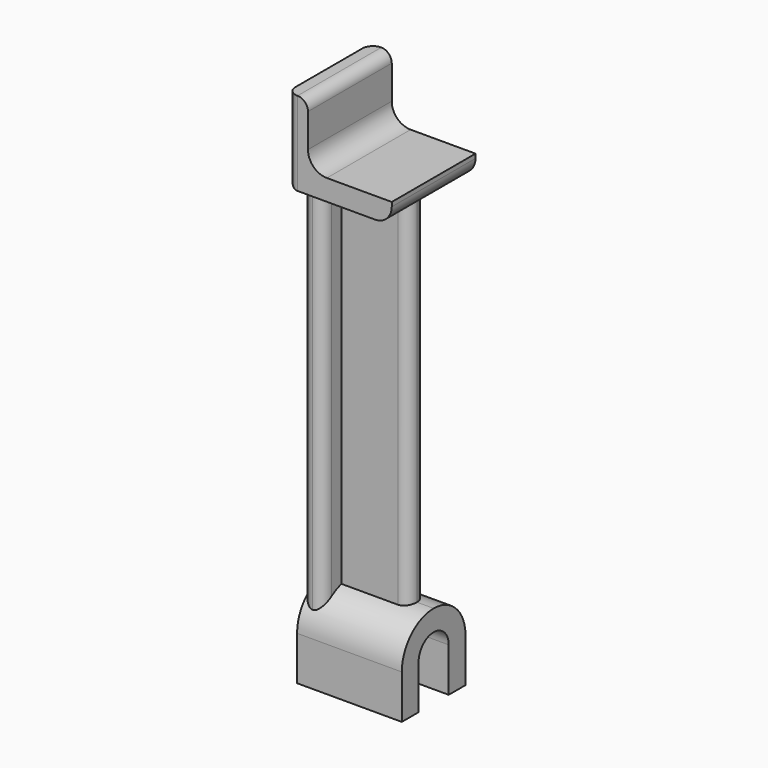
from build123d import *

# Parameters (mm, degrees)
F1_DEPTH = 12.5
F3_DEPTH = 25
F4_W     = 16
F4_H     = 5
F5_DEPTH = 89.876524617
F6_R     = 3.99999
F7_R     = 2.4999


# Not quite as in the source:
# - a fillet or chamfer is up to 0.001 mm smaller than in the source, because OpenCascade refuses the exact size


with BuildPart() as f1:
    # F0 (on Front) → F1 (new body, symmetric)
    with BuildSketch(Plane.XZ):
        with BuildLine():
            ThreePointArc((0, 100), (-3.1819805153, 101.3180194847), (-4.5, 104.5))
            Line((-4.5, 104.5), (-4.5, 115))
            Line((-4.5, 115), (-9.5, 115))
            Line((-9.5, 115), (-9.5, 95))
            Line((-9.5, 95), (15.5, 95))
            Line((15.5, 95), (15.5, 100))
            Line((15.5, 100), (0, 100))
        make_face()
    extrude(amount=F1_DEPTH, both=True)



with BuildPart() as f3:
    # F2 (on face) → F3 (new body)
    with BuildSketch(Plane(origin=(-9.5, 0, 0), x_dir=(0, -1, 0), z_dir=(-1, 0, 0))):
        with BuildLine():
            ThreePointArc((-4.5, 0), (0, 4.5), (4.5, 0))
            Line((4.5, 0), (4.5, -10.5))
            Line((4.5, -10.5), (9.5, -10.5))
            Line((9.5, -10.5), (9.5, 0))
            ThreePointArc((9.5, 0), (6.7175144213, 6.7175144213), (0, 9.5))
            ThreePointArc((0, 9.5), (-6.7175144213, 6.7175144213), (-9.5, 0))
            Line((-9.5, 0), (-9.5, -10.5))
            Line((-9.5, -10.5), (-4.5, -10.5))
            Line((-4.5, -10.5), (-4.5, 0))
        make_face()
    extrude(amount=-F3_DEPTH)


with BuildPart() as f1_1:
    add(f1.part)

    add(f3.part)  # F5 merges F3
    # F4 (on face) → F5 (join, through all)
    with BuildSketch(Plane(origin=(0, 0, 95), x_dir=(1, 0, 0), z_dir=(0, 0, -1))):
        Polygon((-4.5, 8), (-9.5, 8), (-9.5, -8), (-4.5, -8), (-4.5, -2.5), (-4.5, 2.5), align=None)
        with Locations((3.5, 0)):
            Rectangle(F4_W, F4_H)
    extrude(amount=F5_DEPTH)

    # F6 (radius 4 in the source; OpenCascade refuses exactly that, so slightly less here)
    f6_edges = [f1_1.edges().sort_by_distance(p)[0] for p in [
        (15.5, 0, 95),
    ]]
    fillet(f6_edges, radius=F6_R)

    # F7 (radius 2.5 in the source; OpenCascade refuses exactly that, so slightly less here)
    f7_edges = [f1_1.edges().sort_by_distance(p)[0] for p in [
        (11.5, -2.5, 52.082576),
        (11.5, 2.5, 52.082576),
        (-4.5, -8, 50.061738),
        (-4.5, 8, 50.061738),
        (-9.5, 8, 50.061738),
        (-9.5, -8, 50.061738),
        (-9.5, -10.25, 95),
        (-9.5, 10.25, 95),
        (-9.5, -12.5, 105),
        (-9.5, 12.5, 105),
        (-4.5, 0, 115),
    ]]
    fillet(f7_edges, radius=F7_R)


solid = f1_1.part
